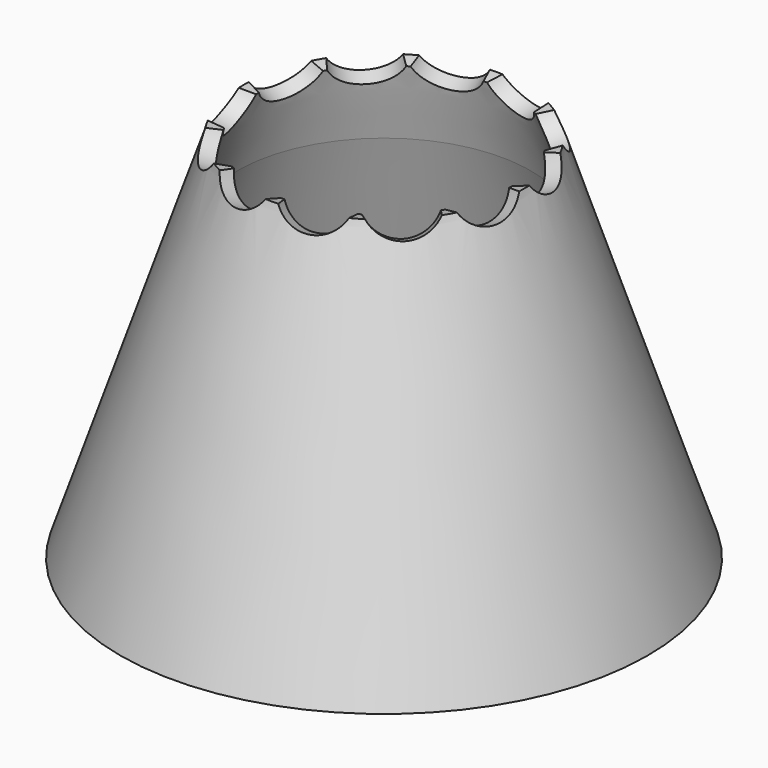
from build123d import *

# Parameters (mm, degrees)
F2_ANGLE = 30
F7_R     = 34.5
F8_DEPTH = 50
F9_COUNT = 12


with BuildPart() as f2:
    # F0 (on Front) → F2 (revolve)
    with BuildSketch(Plane.XZ):
        Polygon((-250, 0), (-150, 300), (-128.5085546445, 379.4732062371), (-143.5085546445, 379.4732062371), (-270, 0), align=None)
    revolve(axis=Axis((0, 0, 153.8413912058), (0, 0, 1)), revolution_arc=F2_ANGLE)

    # F7 (on face) → F8 (cut, symmetric)
    with BuildSketch(Plane(origin=(-236.5949971263, -63.3954384132, 89.1512931807), x_dir=(0.2275892479, -0.9699735704, -0.0857578394), z_dir=(-0.9076733712, -0.2432103468, 0.3420201433))):
        with Locations((-29.5747305444, 322.5639681518)):
            Circle(F7_R)
    extrude(amount=F8_DEPTH, both=True, mode=Mode.SUBTRACT)

    # F9: F2 ×12 about axis
    f9_axis = Axis((0, 0, 153.8413912058), (0, 0, 1))


with BuildPart() as f2_1:
    add(f2.part)
    for i in range(1, F9_COUNT):
        add(f2.part.rotate(f9_axis, i * 360 / F9_COUNT))

    # F10 (on Front) → F11 (revolve, cut)
    with BuildSketch(Plane.XZ):
        Polygon((-155.5699557066, 382.1136057377), (-88.8577103615, 366.885393858), (-68.5985766833, 451.6429048999), (-222.9030430317, 443.2130157948), align=None)
    revolve(axis=Axis((0, 0, 153.8413912058), (0, 0, 1)), mode=Mode.SUBTRACT)


solid = f2_1.part
